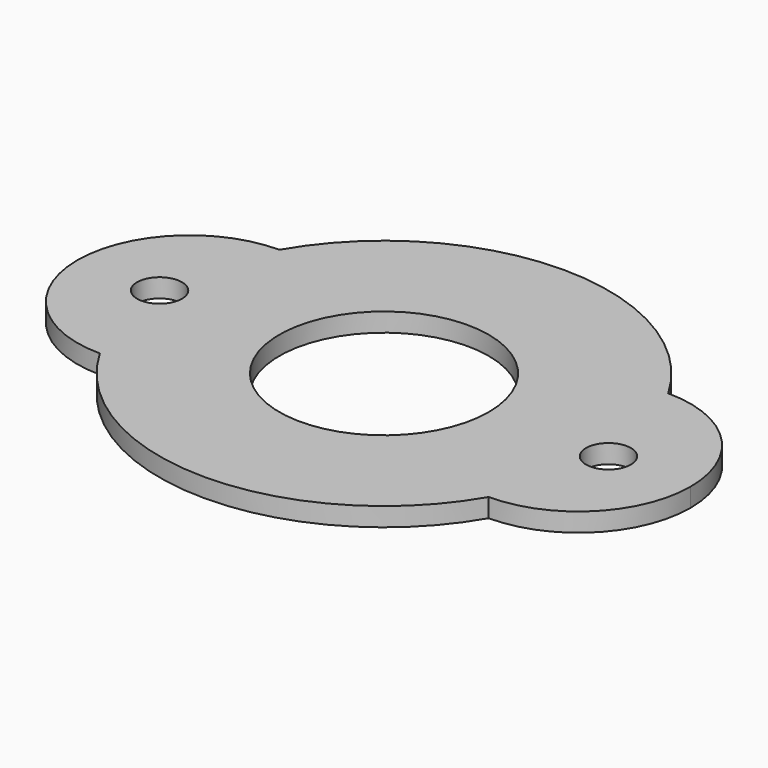
from build123d import *

# Parameters (mm, degrees)
F0_R     = 7
F1_DEPTH = 1.25
F2_R     = 7.49999
F3_D     = 3


# Not quite as in the source:
# - a fillet or chamfer is up to 0.001 mm smaller than in the source, because OpenCascade refuses the exact size


with BuildPart() as f1:
    # F0 (on Top) → F1 (new body)
    with BuildSketch(Plane.XY):
        with BuildLine():
            ThreePointArc((-12.990381, -7.5), (-15, 0), (-12.990381, 7.5))
            Line((-12.990381, 7.5), (-20.490381, 7.5))
            Line((-20.490381, 7.5), (-20.490381, -7.5))
            Line((-20.490381, -7.5), (-12.990381, -7.5))
        make_face()
        with BuildLine():
            ThreePointArc((12.990381, -7.5), (14.488887, -3.882286), (15, 0))
            ThreePointArc((15, 0), (14.488887, 3.882286), (12.990381, 7.5))
            ThreePointArc((12.990381, 7.5), (0, 15), (-12.990381, 7.5))
            ThreePointArc((-12.990381, 7.5), (-15, 0), (-12.990381, -7.5))
            ThreePointArc((-12.990381, -7.5), (0, -15), (12.990381, -7.5))
        make_face()
        Circle(F0_R, mode=Mode.SUBTRACT)
        with BuildLine():
            ThreePointArc((12.990381, 7.5), (14.488887, 3.882286), (15, 0))
            ThreePointArc((15, 0), (14.488887, -3.882286), (12.990381, -7.5))
            Line((12.990381, -7.5), (20.490381, -7.5))
            Line((20.490381, -7.5), (20.490381, 7.5))
            Line((20.490381, 7.5), (12.990381, 7.5))
        make_face()
    extrude(amount=F1_DEPTH)

    # F2 (radius 7.5 in the source; OpenCascade refuses exactly that, so slightly less here)
    f2_edges = [f1.edges().sort_by_distance(p)[0] for p in [
        (-20.490381, 7.5, 0.625),
        (-20.490381, -7.5, 0.625),
        (20.490381, 7.5, 0.625),
        (20.490381, -7.5, 0.625),
    ]]
    fillet(f2_edges, radius=F2_R)

    # F3 (through all)
    with Locations(Plane(origin=(0, 0, 0), x_dir=(1, 0, 0), z_dir=(0, 0, -1))):
        with Locations((15, 0), (-15, 0)):
            Hole(F3_D / 2)


solid = f1.part
